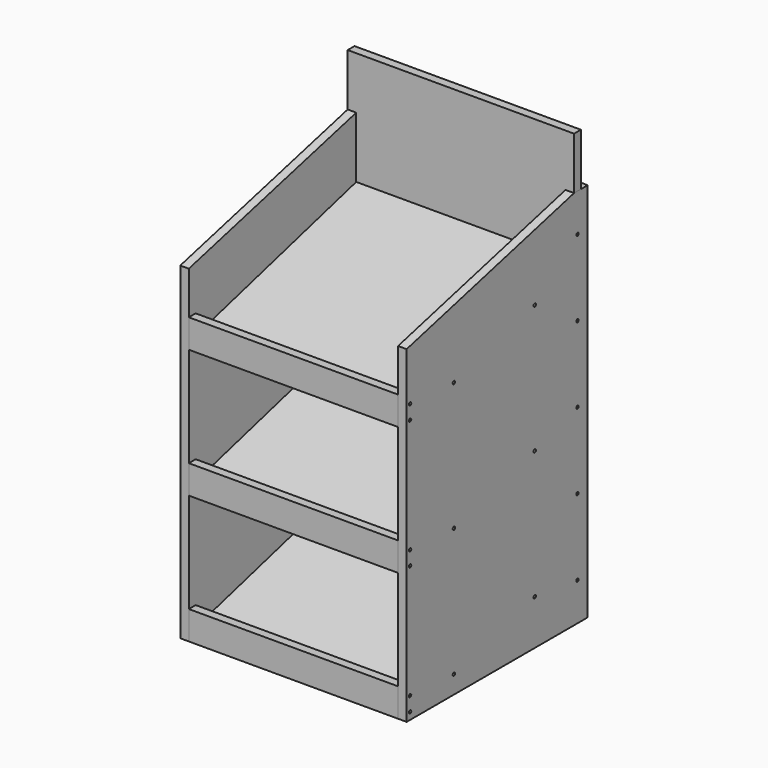
from build123d import *

# Parameters (mm, degrees)
F0_W      = 9
F0_H      = 400
F1_DEPTH  = 238
F3_DEPTH  = 10
F4_R      = 1.5875
F5_DEPTH  = 9
F6_R      = 1.5875
F7_DEPTH  = 25
F9_W      = 220
F9_H      = 9
F10_DEPTH = 400
F11_W     = 9
F11_H     = 9
F11_W_2   = 220
F12_DEPTH = 55
F13_R     = 1.5875
F14_DEPTH = 220
F15_DEPTH = 220


# Not quite as in the source:
# - a feature names something its author has since deleted; it is built from what else it names


with BuildPart() as f1:
    # F0 (on Front) → F1 (new body)
    with BuildSketch(Plane.XZ):
        with Locations((-114.5, 35)):
            Rectangle(F0_W, F0_H)
    extrude(amount=F1_DEPTH)

    # F2 (on face) → F3 (cut)
    with BuildSketch(Plane(origin=(-119, 0, 0), x_dir=(0, -1, 0), z_dir=(-1, 0, 0))):
        Polygon((238, 180), (238, 235), (18, 235), align=None)
    extrude(amount=-F3_DEPTH, mode=Mode.SUBTRACT)

    # F4 (on face) → F5 (cut)
    with BuildSketch(Plane(origin=(-119, 0, 0), x_dir=(0, -1, 0), z_dir=(-1, 0, 0))):
        with Locations((13.5, 195)):
            Circle(F4_R)
        with Locations((13.5, 115)):
            Circle(F4_R)
        with Locations((13.5, 35)):
            Circle(F4_R)
        with Locations((13.5, -45)):
            Circle(F4_R)
        with Locations((13.5, -125)):
            Circle(F4_R)
    extrude(amount=-F5_DEPTH, mode=Mode.SUBTRACT)

    # F6 (on face) → F7 (cut)
    with BuildSketch(Plane.YZ.offset(-110)):
        with Locations((-175.8740795541, -146.1062097075)):
            Circle(F6_R)
        with Locations((-175.8740795541, -11.1062097075)):
            Circle(F6_R)
        with Locations((-175.8740795541, 123.8937902925)):
            Circle(F6_R)
        with Locations((-69.6222386623, 152.3638852538)):
            Circle(F6_R)
        with Locations((-69.6222386623, 17.3638852538)):
            Circle(F6_R)
        with Locations((-69.6222386623, -117.6361147462)):
            Circle(F6_R)
        with Locations((-233.5, -142.5)):
            Circle(F6_R)
        with Locations((-233.5, -157.5)):
            Circle(F6_R)
        with Locations((-233.5, -7.5)):
            Circle(F6_R)
        with Locations((-233.5, -22.5)):
            Circle(F6_R)
        with Locations((-233.5, 127.5)):
            Circle(F6_R)
        with Locations((-233.5, 112.5)):
            Circle(F6_R)
    extrude(amount=-F7_DEPTH, mode=Mode.SUBTRACT)


with BuildPart() as f8_1:
    # F8: instance of F1
    add(f1.part.mirror(Plane.YZ))


with BuildPart() as f10:
    # F9 (on face) → F10 (new body)
    with BuildSketch(Plane(origin=(0, 0, -165), x_dir=(1, 0, 0), z_dir=(0, 0, -1))):
        with Locations((0, 13.5)):
            Rectangle(F9_W, F9_H)
    extrude(amount=-F10_DEPTH)

    # F11 (on face) → F12 (join)
    with BuildSketch(Plane.XY.offset(235)):
        with Locations((114.5, -13.5)):
            Rectangle(F11_W, F11_H)
        with Locations((0, -13.5)):
            Rectangle(F11_W_2, F11_H)
        with Locations((-114.5, -13.5)):
            Rectangle(F11_W, F11_H)
    extrude(amount=F12_DEPTH)


with BuildPart() as f14:
    # F13 (on face) → F14 (new body)
    with BuildSketch(Plane.YZ.offset(-110)):
        Polygon((-238, -135), (-238, -165), (-229, -165), (-229, -155.6825143763), (-229, -135), align=None)
        with Locations((-233.5, -157.5)):
            Circle(F13_R, mode=Mode.SUBTRACT)
        with Locations((-233.5, -142.5)):
            Circle(F13_R, mode=Mode.SUBTRACT)
    extrude(amount=F14_DEPTH)


with BuildPart() as f14b:
    # F13 (on face) → F14, piece 2 (new body)
    with BuildSketch(Plane.YZ.offset(-110)):
        Polygon((-238, 0), (-238, -30), (-229, -30), (-229, -20.6825143763), (-229, 0), align=None)
        with Locations((-233.5, -22.5)):
            Circle(F13_R, mode=Mode.SUBTRACT)
        with Locations((-233.5, -7.5)):
            Circle(F13_R, mode=Mode.SUBTRACT)
    extrude(amount=F14_DEPTH)


with BuildPart() as f14c:
    # F13 (on face) → F14, piece 3 (new body)
    with BuildSketch(Plane.YZ.offset(-110)):
        Polygon((-238, 135), (-238, 105), (-229, 105), (-229, 114.3174856237), (-229, 135), align=None)
        with Locations((-233.5, 112.5)):
            Circle(F13_R, mode=Mode.SUBTRACT)
        with Locations((-233.5, 127.5)):
            Circle(F13_R, mode=Mode.SUBTRACT)
    extrude(amount=F14_DEPTH)


with BuildPart() as f15:
    # F13 (on face) → F15 (new body)
    with BuildSketch(Plane.YZ.offset(-110)):
        Polygon((-229, 114.3174856237), (-229, 105), (-18, 161.537279603), (-18, 170.8547652267), align=None)
        with Locations((-175.8740795541, 123.8937902925)):
            Circle(F13_R, mode=Mode.SUBTRACT)
        with Locations((-69.6222386623, 152.3638852538)):
            Circle(F13_R, mode=Mode.SUBTRACT)
    extrude(amount=F15_DEPTH)


with BuildPart() as f15b:
    # F13 (on face) → F15, piece 2 (new body)
    with BuildSketch(Plane.YZ.offset(-110)):
        Polygon((-229, -20.6825143763), (-229, -30), (-18, 26.537279603), (-18, 35.8547652267), align=None)
        with Locations((-175.8740795541, -11.1062097075)):
            Circle(F13_R, mode=Mode.SUBTRACT)
        with Locations((-69.6222386623, 17.3638852538)):
            Circle(F13_R, mode=Mode.SUBTRACT)
    extrude(amount=F15_DEPTH)


with BuildPart() as f15c:
    # F13 (on face) → F15, piece 3 (new body)
    with BuildSketch(Plane.YZ.offset(-110)):
        Polygon((-229, -155.6825143763), (-229, -165), (-18, -108.462720397), (-18, -99.1452347733), align=None)
        with Locations((-175.8740795541, -146.1062097075)):
            Circle(F13_R, mode=Mode.SUBTRACT)
        with Locations((-69.6222386623, -117.6361147462)):
            Circle(F13_R, mode=Mode.SUBTRACT)
    extrude(amount=F15_DEPTH)


solid = Compound([f1.part, f8_1.part, f10.part, f14.part, f14b.part, f14c.part, f15.part, f15b.part, f15c.part])
